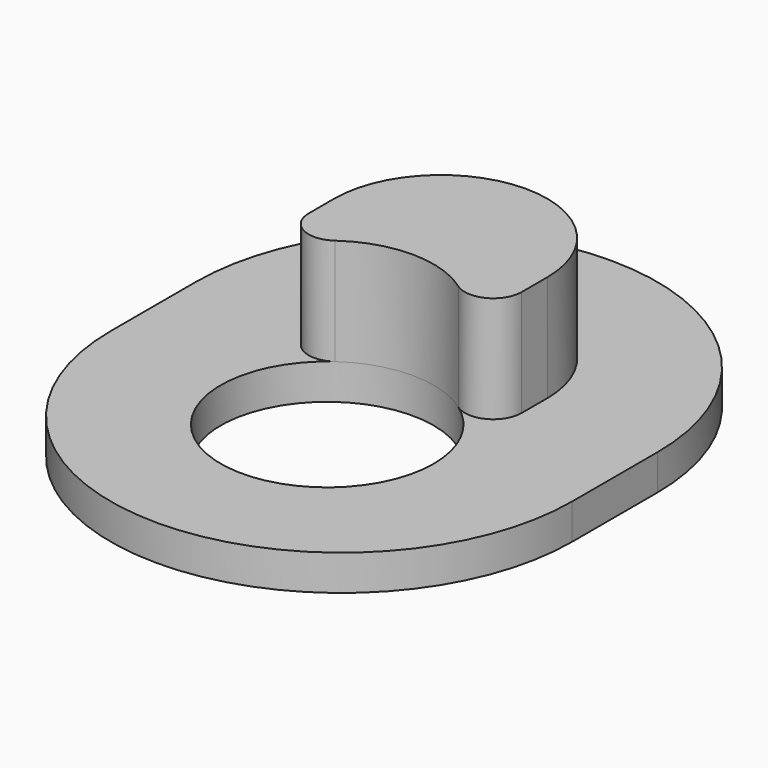
from build123d import *
from build123d import SkipClean  # not in build123d's __all__

# Parameters (mm, degrees)
F0_R        = 4.7625
F1_DEPTH    = 1.5875
F3_DEPTH    = 4.7625
F4_T1_DEPTH = 17.0592221242


# Not quite as in the source:
# - a fillet or chamfer that OpenCascade refuses, or shapes differently, is made with other operations: its cross-section is extruded or revolved along the edge and cut away or added


with BuildPart() as f1:
    # F0 (on Top) → F1 (new body)
    with BuildSketch(Plane.XY):
        with BuildLine():
            Line((-10.31875, 4.7625), (-10.31875, 0))
            ThreePointArc((-10.31875, 0), (0, -10.31875), (10.31875, 0))
            Line((10.31875, 0), (10.31875, 4.7625))
            ThreePointArc((10.31875, 4.7625), (0, 15.08125), (-10.31875, 4.7625))
        make_face()
        with Locations((0, -0.79375)):
            Circle(F0_R, mode=Mode.SUBTRACT)
    extrude(amount=F1_DEPTH)

    # F2 (on face) → F3 (join)
    with BuildSketch(Plane.XY.offset(1.5875)):
        with BuildLine():
            ThreePointArc((-4.7625, -0.79375), (0, 3.96875), (4.7625, -0.79375))
            Line((4.7625, -0.79375), (4.7625, 5.55625))
            ThreePointArc((4.7625, 5.55625), (0, 10.31875), (-4.7625, 5.55625))
            Line((-4.7625, 5.55625), (-4.7625, -0.79375))
        make_face()
    with SkipClean():  # cleaning this boolean's faces spoils the solid; the shape is the same uncleaned
        extrude(amount=F3_DEPTH)

    # F4: fillet of radius 1.27 on 2 edges, made by hand

    # F4_s2 → F4_t1 (cut)
    with BuildSketch(Plane.XY.offset(1.5875)):
        with BuildLine():
            ThreePointArc((4.7625, 4.1249388497), (4.075215964, 2.9965142376), (2.7572368421, 3.0894254076))
            ThreePointArc((2.7572368421, 3.0894254076), (4.2315922955, 1.3914348651), (4.7625, -0.79375))
            Line((4.7625, -0.79375), (4.7625, 4.1249388497))
        make_face()
        with BuildLine():
            ThreePointArc((-4.7625, 4.1249388497), (-4.075215964, 2.9965142376), (-2.7572368421, 3.0894254076))
            ThreePointArc((-2.7572368421, 3.0894254076), (-4.2315922955, 1.3914348651), (-4.7625, -0.79375))
            Line((-4.7625, -0.79375), (-4.7625, 4.1249388497))
        make_face()
    extrude(amount=F4_T1_DEPTH, mode=Mode.SUBTRACT)


solid = f1.part
